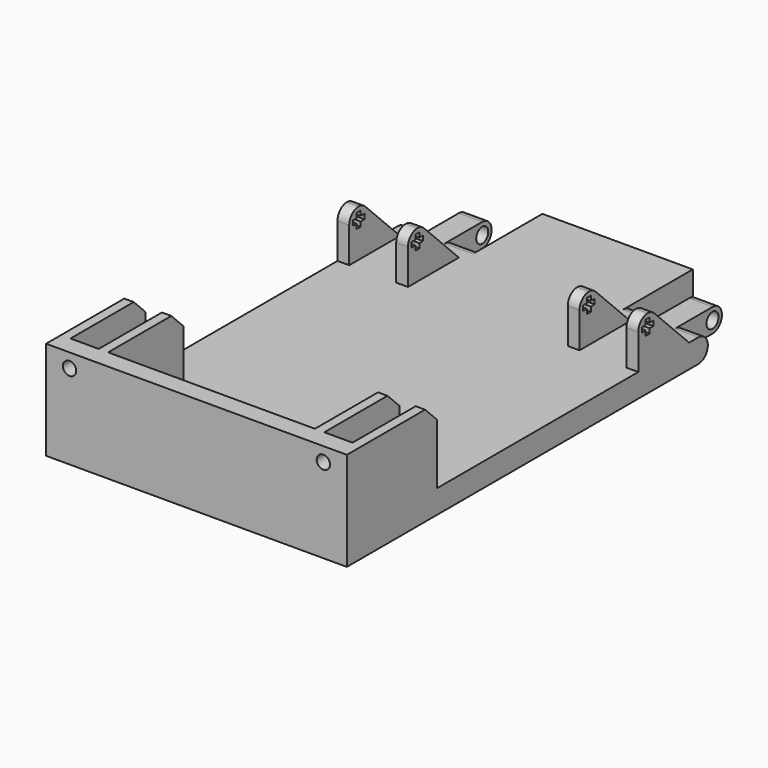
from build123d import *

# Parameters (mm, degrees)
F1_DEPTH  = 7.9375
F2_R      = 3.96874
F3_R      = 2.54
F4_DEPTH  = 25.4
F5_R      = 2.54
F6_DEPTH  = 7.9375
F7_W      = 3.96875
F7_H      = 25.4
F8_DEPTH  = 15.875
F9_W      = 1.6891
F9_H      = 1.56845
F9_H_2    = 1.6891
F9_W_2    = 1.56845
F10_DEPTH = 101.6
F12_DEPTH = 25.4
F13_SIZE  = 5.08
F14_R     = 2.2479
F15_DEPTH = 6.35


# Not quite as in the source:
# - a fillet or chamfer is up to 0.001 mm smaller than in the source, because OpenCascade refuses the exact size
# - an extrude ends at something that could not be found from the text; its depth is read off the source's solid


with BuildPart() as f1:
    # F0 (on Top) → F1 (new body)
    with BuildSketch(Plane.XY):
        Polygon((0, 152.4), (0, 0), (101.6, 0), (101.6, 152.4), (93.6625, 152.4), (93.6625, 168.275), (85.725, 168.275), (85.725, 152.4), (76.2, 152.4), (76.2, 177.8), (25.4, 177.8), (25.4, 152.4), (15.875, 152.4), (15.875, 168.275), (7.9375, 168.275), (7.9375, 152.4), align=None)
    extrude(amount=F1_DEPTH)

    # F2 (radius 3.96875 in the source; OpenCascade refuses exactly that, so slightly less here)
    f2_edges = [f1.edges().sort_by_distance(p)[0] for p in [
        (20.6375, 152.4, 0),
        (20.6375, 152.4, 7.9375),
        (11.90625, 168.275, 0),
        (11.90625, 168.275, 7.9375),
        (3.96875, 152.4, 0),
        (3.96875, 152.4, 7.9375),
        (80.9625, 152.4, 7.9375),
        (80.9625, 152.4, 0),
        (97.63125, 152.4, 0),
        (97.63125, 152.4, 7.9375),
        (89.69375, 168.275, 7.9375),
        (89.69375, 168.275, 0),
    ]]
    fillet(f2_edges, radius=F2_R)

    # F3 (on face) → F4 (cut, through all)
    with BuildSketch(Plane(origin=(0, 0, 0), x_dir=(0, -1, 0), z_dir=(-1, 0, 0))):
        with Locations((-164.30625, 3.96875)):
            Circle(F3_R)
    extrude(amount=-F4_DEPTH, mode=Mode.SUBTRACT)

    # F5 (on face) → F6 (cut, through all)
    with BuildSketch(Plane.YZ.offset(93.6625)):
        with Locations((164.30625, 3.96875)):
            Circle(F5_R)
    extrude(amount=-F6_DEPTH, mode=Mode.SUBTRACT)

    # F7 (on face) → F8 (join)
    with BuildSketch(Plane.XY.offset(7.9375)):
        with Locations((1.984375, 135.73125)):
            Rectangle(F7_W, F7_H)
        with Locations((21.828125, 135.73125)):
            Rectangle(F7_W, F7_H)
        with Locations((99.615625, 135.73125)):
            Rectangle(F7_W, F7_H)
        with Locations((79.771875, 135.73125)):
            Rectangle(F7_W, F7_H)
    extrude(amount=F8_DEPTH)

    # F9 (on face) → F10 (cut, through all)
    with BuildSketch(Plane(origin=(0, 0, 0), x_dir=(0, -1, 0), z_dir=(-1, 0, 0))):
        with BuildLine():
            Line((-123.03125, 19.84375), (-123.03125, 23.8125))
            Line((-123.03125, 23.8125), (-127, 23.8125))
            ThreePointArc((-127, 23.8125), (-124.1936699622, 22.6500800378), (-123.03125, 19.84375))
        make_face()
        with BuildLine():
            ThreePointArc((-129.8063300378, 22.6500800378), (-128.5187748722, 23.5103968947), (-127, 23.8125))
            Line((-127, 23.8125), (-148.43125, 23.8125))
            Line((-148.43125, 23.8125), (-148.43125, 7.9375))
            Line((-148.43125, 7.9375), (-144.5189100757, 7.9375))
            Line((-144.5189100757, 7.9375), (-129.8063300378, 22.6500800378))
        make_face()
        with Locations((-127, 18.214975)):
            Rectangle(F9_W, F9_H)
        with Locations((-127, 19.84375)):
            Rectangle(F9_W, F9_H_2)
        with Locations((-125.371225, 19.84375)):
            Rectangle(F9_W_2, F9_H_2)
        with Locations((-127, 21.472525)):
            Rectangle(F9_W, F9_H)
        with Locations((-128.628775, 19.84375)):
            Rectangle(F9_W_2, F9_H_2)
    extrude(amount=-F10_DEPTH, mode=Mode.SUBTRACT)

    # F11 (on face) → F12 (join)
    with BuildSketch(Plane.XY.offset(7.9375)):
        Polygon((0, 38.1), (0, 0), (101.6, 0), (101.6, 38.1), (98.425, 38.1), (98.425, 6.35), (88.9, 6.35), (88.9, 38.1), (85.725, 38.1), (85.725, 6.35), (15.875, 6.35), (15.875, 38.1), (12.7, 38.1), (12.7, 6.35), (3.175, 6.35), (3.175, 38.1), align=None)
    extrude(amount=F12_DEPTH)

    # F13
    f13_edges = [f1.edges().sort_by_distance(p)[0] for p in [
        (14.2875, 38.1, 33.3375),
        (1.5875, 38.1, 33.3375),
        (87.3125, 38.1, 33.3375),
        (100.0125, 38.1, 33.3375),
    ]]
    chamfer(f13_edges, length=F13_SIZE)

    # F14 (on face) → F15 (cut, through all)
    with BuildSketch(Plane.XZ):
        with Locations((93.6625, 28.575)):
            Circle(F14_R)
        with Locations((7.9375, 28.575)):
            Circle(F14_R)
    extrude(amount=-F15_DEPTH, mode=Mode.SUBTRACT)


solid = f1.part
